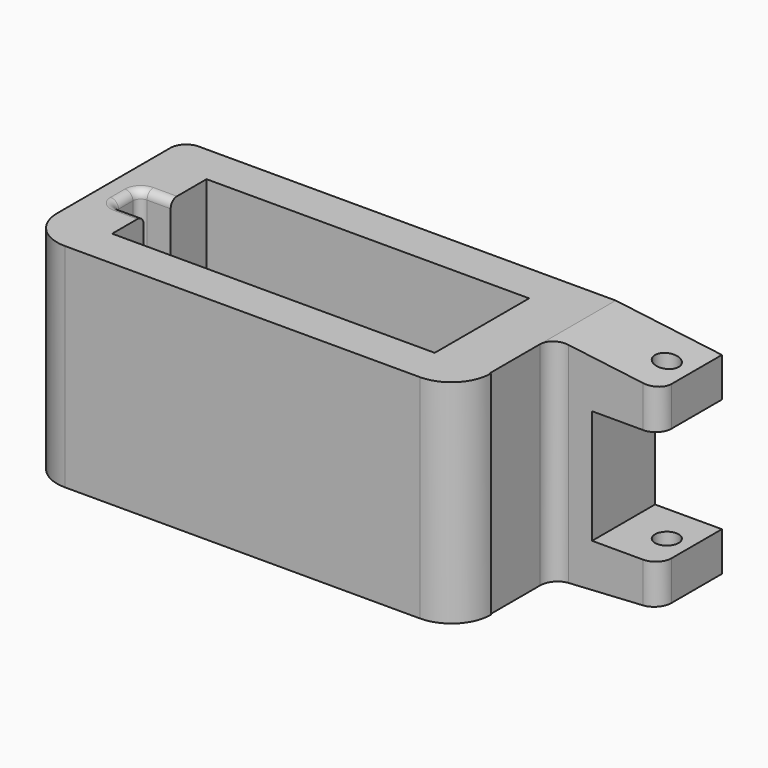
from build123d import *

# Parameters (mm, degrees)
F0_W           = 41
F0_H           = 27
F1_DEPTH       = 5
F0_W_2         = 7
F2_DEPTH       = 20
F3_DEPTH       = 20
F4_DEPTH       = 10
F5_R           = 2
F8_D           = 3
F8_DEPTH       = 12
F8_TIP         = 0.9012909285
F8_ON_F6_D     = 3
F8_ON_F6_DEPTH = 12
F8_ON_F6_TIP   = 0.9012909285
F9_W           = 48.1226687921
F9_H           = 27
F9_W_2         = 55.1226687921
F10_DEPTH      = 5
F11_R          = 4.99999
F12_W          = 4.2837616056
F12_H          = 27.1169293898
F13_DEPTH      = 4
F14_F1_R       = 1
F14_F2_R       = 1
F15_R          = 1


# Not quite as in the source:
# - a fillet or chamfer is up to 0.001 mm smaller than in the source, because OpenCascade refuses the exact size


with BuildPart() as f1:
    # F0 (on Front) → F1 (new body)
    with BuildSketch(Plane.XZ):
        with Locations((-0.1147079957, -0.1861773429)):
            Rectangle(F0_W, F0_H)
    extrude(amount=F1_DEPTH)

    # F0 (on Front) → F2 (join)
    with BuildSketch(Plane.XZ):
        with Locations((23.8852920043, -0.1861773429)):
            Rectangle(F0_W_2, F0_H)
    extrude(amount=F2_DEPTH)

    # F0 (on Front) → F3 (join)
    with BuildSketch(Plane.XZ):
        with Locations((-24.1147079957, -0.1861773429)):
            Rectangle(F0_W_2, F0_H)
    extrude(amount=F3_DEPTH)

    # F0 (on Front) → F4 (join)
    with BuildSketch(Plane.XZ):
        Polygon((40.8852920043, 11.6193783459), (27.3852920043, 13.3138226571), (27.3852920043, -13.6861773429), (40.8852920043, -12.8806216541), (40.8852920043, -7.8806216541), (32.3852920043, -7.8806216541), (32.3852920043, 6.6193783459), (40.8852920043, 6.6193783459), align=None)
    extrude(amount=F4_DEPTH)

    # F5
    f5_edges = [f1.edges().sort_by_distance(p)[0] for p in [
        (27.385292, -10, -0.186177),
        (-27.614708, 0, -0.186177),
        (40.885292, -10, -10.380622),
        (40.885292, -10, 9.119378),
    ]]
    fillet(f5_edges, radius=F5_R)

    # F8 (one way)
    with BuildSketch(Plane(origin=(0, 0, 6.6193783459), x_dir=(1, 0, 0), z_dir=(0, 0, -1))):
        with Locations((37.8852920043, 5)):
            Circle(F8_D / 2)
    extrude(amount=-F8_DEPTH, mode=Mode.SUBTRACT)
    with Locations(Plane(origin=(0, 0, 6.6193783459), x_dir=(1, 0, 0), z_dir=(0, 0, -1))):
        with Locations((37.8852920043, 5)):
            with Locations((0, 0, -(F8_DEPTH + F8_TIP / 2))):  # 118° drill point
                Cone(0, F8_D / 2, F8_TIP, mode=Mode.SUBTRACT)

    # F8 on F6 (one way)
    with BuildSketch(Plane.XY.offset(-7.8806216541)):
        with Locations((37.8852920043, -5)):
            Circle(F8_ON_F6_D / 2)
    extrude(amount=-F8_ON_F6_DEPTH, mode=Mode.SUBTRACT)
    with Locations(Plane.XY.offset(-7.8806216541)):
        with Locations((37.8852920043, -5)):
            with Locations((0, 0, -(F8_ON_F6_DEPTH + F8_ON_F6_TIP / 2))):  # 118° drill point
                Cone(0, F8_ON_F6_D / 2, F8_ON_F6_TIP, mode=Mode.SUBTRACT)

    # F9 (on face) → F10 (join)
    with BuildSketch(Plane.XZ.offset(20)):
        with Locations((3.4466264003, -0.1861773429)):
            Rectangle(F9_W, F9_H)
        with Locations((-0.0533735997, -0.1861773429)):
            Rectangle(F9_W_2, F9_H)
    extrude(amount=F10_DEPTH)

    # F11 (radius 5 in the source; OpenCascade refuses exactly that, so slightly less here)
    f11_edges = [f1.edges().sort_by_distance(p)[0] for p in [
        (27.507961, -25, -0.186177),
        (-27.614708, -25, -0.186177),
    ]]
    fillet(f11_edges, radius=F11_R)

    # F12 (on face) → F13 (cut)
    with BuildSketch(Plane.YZ.offset(-20.6147079957)):
        with Locations((-12.8439003602, -0.2446420378)):
            Rectangle(F12_W, F12_H)
    extrude(amount=-F13_DEPTH, mode=Mode.SUBTRACT)

    # F14: fillet of radius 1 on 3 edges, made by hand

    # F14_f1
    f14_f1_edges = [f1.edges().sort_by_distance(p)[0] for p in [
        (-24.6147079957, -14.985781163, -0.1861773429),
        (-24.6147079957, -10.7020195574, -0.1861773429),
    ]]
    fillet(f14_f1_edges, radius=F14_F1_R)

    # F14_f2
    f14_f2_edges = [f1.edges().sort_by_distance(p)[0] for p in [
        (-24.6147079957, -12.8439003602, 13.3138226571),
        (-24.3218147769, -10.9949127762, 13.3138226571),
        (-24.3218147769, -14.6928879442, 13.3138226571),
    ]]
    fillet(f14_f2_edges, radius=F14_F2_R)

    # F15
    f15_edges = [f1.edges().sort_by_distance(p)[0] for p in [
        (-22.114708, -14.985781, -13.686177),
        (-22.114708, -10.70202, -13.686177),
        (-24.321815, -10.994913, -13.686177),
        (-24.614708, -12.8439, -13.686177),
        (-24.321815, -14.692888, -13.686177),
    ]]
    fillet(f15_edges, radius=F15_R)


solid = f1.part
